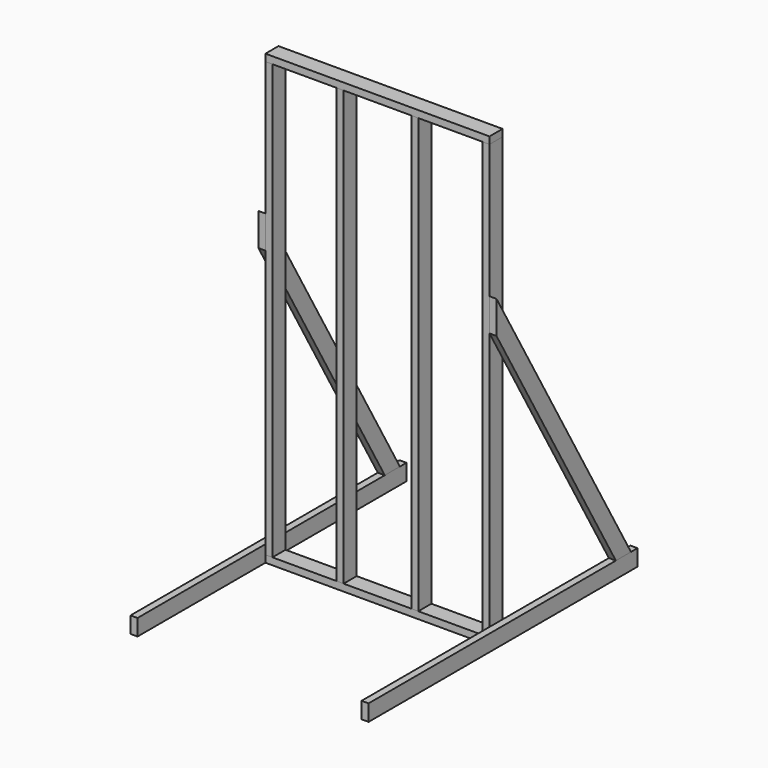
from build123d import *

# Parameters (mm, degrees)
F0_W      = 38.1
F0_H      = 2362.2
F1_DEPTH  = 88.9
F5_W      = 1219.2
F5_H      = 38.1
F6_DEPTH  = 88.9
F8_W      = 1828.8
F8_H      = 88.9
F9_DEPTH  = 38.1
F12_DEPTH = 38.1
F14_W     = 1981.2
F14_H     = 88.9
F15_DEPTH = 38.1
F20_DEPTH = 38.1


# Not quite as in the source:
# - a feature of the source that left no trace in its solid (it failed there, or was rolled back) is left out
# - a pattern or mirror of a feature is missing from the dataset's text; its kind, count and spacing are read off the source's solid


with BuildPart() as f1:
    # F0 (on Front) → F1 (new body)
    with BuildSketch(Plane.XZ):
        with Locations((19.05, 1181.1)):
            Rectangle(F0_W, F0_H)
    extrude(amount=F1_DEPTH)


with BuildPart() as f2_1:
    # F2: copy of F1
    add(f1.part.moved(Location((387.35, 0, 0))))


with BuildPart() as f3_1:
    # F3: copy of F2_1
    add(f2_1.part.moved(Location((406.4, 0, 0))))


with BuildPart() as f4_1:
    # F4: copy of F3_1
    add(f3_1.part.moved(Location((387.35, 0, 0))))


with BuildPart() as f6:
    # F5 (on Front) → F6 (new body)
    with BuildSketch(Plane.XZ):
        with Locations((609.6, -19.05)):
            Rectangle(F5_W, F5_H)
    extrude(amount=F6_DEPTH)


with BuildPart() as f6_copies_1:
    # F6_copies: instance of F6
    add(f6.part.mirror(Plane.XY.offset(1181.1)))


with BuildPart() as f9:
    # F8 (on face) → F9 (new body)
    with BuildSketch(Plane(origin=(0, 0, 0), x_dir=(0, -1, 0), z_dir=(-1, 0, 0))):
        with Locations((44.45, 6.35)):
            Rectangle(F8_W, F8_H)
    extrude(amount=F9_DEPTH)


with BuildPart() as f10_1:
    # F10: copy of F9
    add(f9.part.moved(Location((1257.3, 0, 0))))


with BuildPart() as f12:
    # F11 (on face) → F12 (new body)
    with BuildSketch(Plane(origin=(1219.2, 0, 0), x_dir=(0, -1, 0), z_dir=(-1, 0, 0))):
        Polygon((0, 1480.6079416481), (-825.5, 50.8), (-722.8471221381, 50.8), (0, 1302.8079416481), align=None)
        Polygon((88.9, 1634.587258441), (0, 1480.6079416481), (0, 1302.8079416481), (88.9, 1456.787258441), align=None)
    extrude(amount=-F12_DEPTH)


with BuildPart() as f13_1:
    # F13: copy of F12
    add(f12.part.moved(Location((-1257.3, 0, 0))))


with BuildPart() as f15:
    # F14 (on Right) → F15 (new body)
    with BuildSketch(Plane.YZ):
        with Locations((-990.6, 1847.85)):
            Rectangle(F14_W, F14_H)
    extrude(amount=-F15_DEPTH)


with BuildPart() as f16_1:
    # F16: copy of F15
    add(f15.part.moved(Location((1257.3, 0, 0))))


with BuildPart() as f17_1:
    # F17: copy of F15
    add(f15.part.moved(Location((0, 0, -1524))))


with BuildPart() as f18_1:
    # F18: copy of F17_1
    add(f17_1.part.moved(Location((1257.3, 0, 0))))


with BuildPart() as f20:
    # F19 (on face) → F20 (new body)
    with BuildSketch(Plane.YZ.offset(1257.3)):
        Polygon((-1114.616916851, 279.4), (-1900.9370329048, 1930.5238945304), (-1981.2, 1892.3), (-1194.8798839462, 241.1761054696), align=None)
    extrude(amount=F20_DEPTH)


with BuildPart() as f21_1:
    # F21: copy of F20
    add(f20.part.moved(Location((-1333.5, 0, 0))))


solid = Compound([f1.part, f2_1.part, f3_1.part, f4_1.part, f6.part, f6_copies_1.part, f9.part, f10_1.part, f12.part, f13_1.part])
